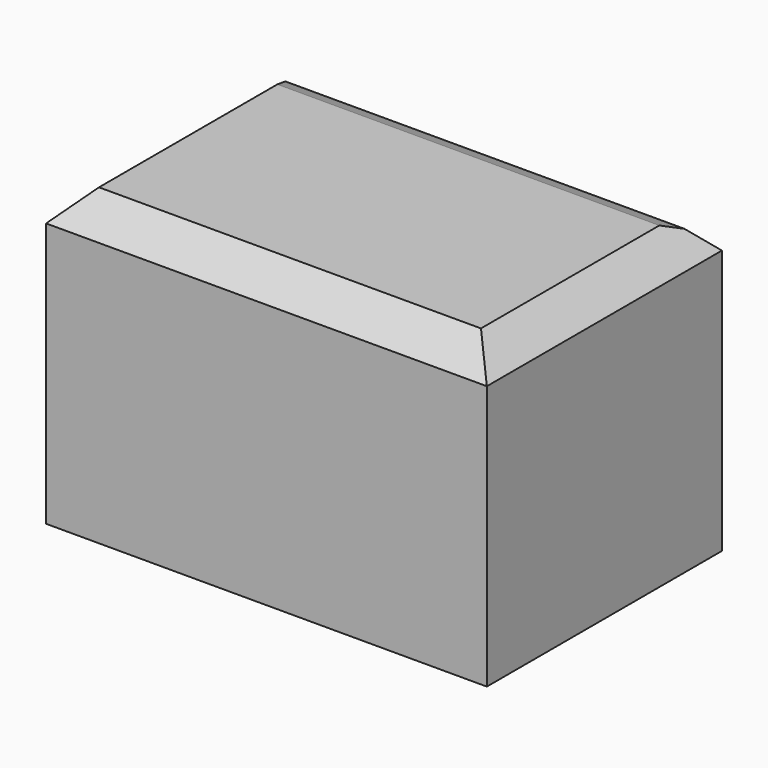
from build123d import *

# Parameters (mm, degrees)
F0_W        = 76.2
F0_H        = 50.8
F1_DEPTH    = 50.8
F2_SIZE     = 5.08
F3_T1_DEPTH = 71.8482991577
F3_T3_DEPTH = 87.6662799398
F3_T5_DEPTH = 102.3282991577


# Not quite as in the source:
# - a fillet or chamfer that OpenCascade refuses, or shapes differently, is made with other operations: its cross-section is extruded or revolved along the edge and cut away or added


with BuildPart() as f1:
    # F0 (on Top) → F1 (new body)
    with BuildSketch(Plane.XY):
        with Locations((19.1995975337, 5.2968291566)):
            Rectangle(F0_W, F0_H)
    extrude(amount=F1_DEPTH)

    # F2
    f2_edges = [f1.edges().sort_by_distance(p)[0] for p in [
        (19.199598, 30.696829, 50.8),
    ]]
    chamfer(f2_edges, length=F2_SIZE)

    # F3: chamfer of 5.08 on 4 edges, made by hand

    # F3_s2 → F3_t1 (cut)
    with BuildSketch(Plane.XZ.offset(-38.6809787354)):
        Polygon((-18.9004024663, 45.72), (-13.8204024663, 50.8), (-18.9004024663, 50.8), align=None)
        Polygon((57.2995975337, 45.72), (52.2195975337, 50.8), (57.2995975337, 50.8), align=None)
    extrude(amount=F3_T1_DEPTH, mode=Mode.SUBTRACT)

    # F3_s4 → F3_t3 (cut)
    with BuildSketch(Plane.YZ.offset(-24.6335424362)):
        Polygon((27.1047267081, 49.3121024484), (23.5126242597, 50.8), (25.6168291566, 50.8), align=None)
    extrude(amount=F3_T3_DEPTH, mode=Mode.SUBTRACT)

    # F3_s6 → F3_t5 (cut)
    with BuildSketch(Plane.YZ.offset(-31.9645520452)):
        Polygon((-15.0231708434, 50.8), (-20.1031708434, 45.72), (-20.1031708434, 50.8), align=None)
    extrude(amount=F3_T5_DEPTH, mode=Mode.SUBTRACT)


solid = f1.part
